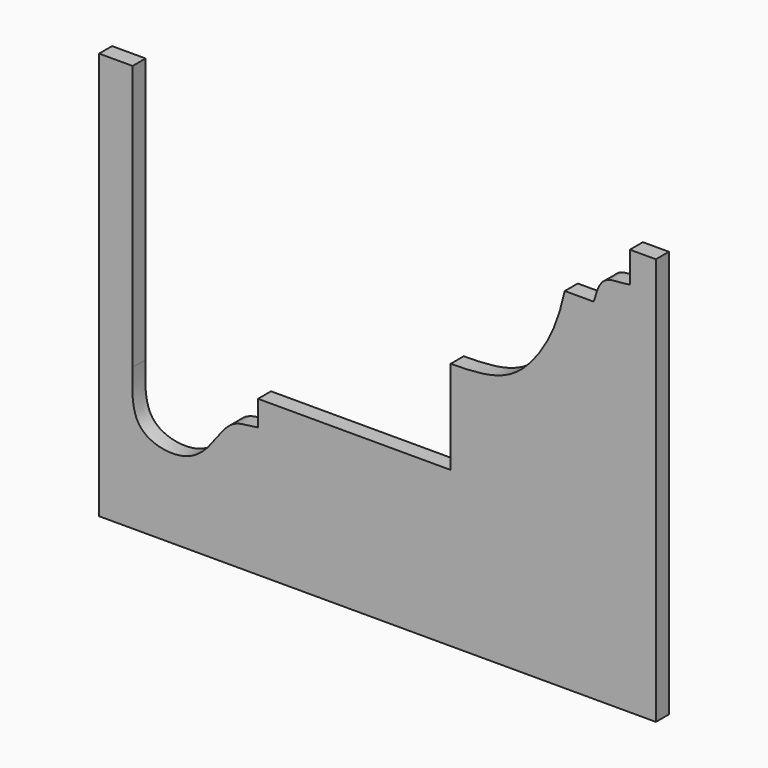
from build123d import *

# Parameters (mm, degrees)
F2_DEPTH = 10


with BuildPart() as f2:
    # F1 (on face) → F2 (new body)
    with BuildSketch(Plane.XZ):
        with BuildLine():
            Line((-91.9840037823, -31.2996767461), (-91.9840037823, 131.8993419409))
            Line((-91.9840037823, 131.8993419409), (-112.6081570983, 131.8993419409))
            Line((-112.6081570983, 131.8993419409), (-112.6081570983, -118.7344565988))
            Line((-112.6081570983, -118.7344565988), (230.0193011761, -118.7344565988))
            Line((230.0193011761, -118.7344565988), (230.0193011761, 131.8993419409))
            Line((230.0193011761, 131.8993419409), (214.0238434076, 131.8993419409))
            Line((214.0238434076, 131.8993419409), (214.0238434076, 113.0083352327))
            add(Edge.make_bspline(
                [(191.6237324476, 96.4869484305), (192.4980250224, 98.1278702864), (193.1536069546, 101.9439997116), (196.1146778047, 108.6562828707), (201.6165341433, 112.5583739062), (211.8606585251, 112.2793213926), (214.0238434076, 113.0083352327)],
                knots=[0, 0, 0, 0, 0.2157210018, 0.4532431975, 0.6893360054, 1, 1, 1, 1], degree=3))
            Line((191.6237324476, 96.4869484305), (173.9649176598, 96.4869484305))
            add(Edge.make_bspline(
                [(173.9649176598, 96.4869484305), (172.0666621983, 87.7106344295), (166.200808661, 67.3071544762), (145.3206230123, 39.4041475495), (121.2131008193, 34.3114486831), (109.1523088398, 34.3117546192), (103.772804141, 34.2541225255)],
                knots=[0, 0, 0, 0, 0.2707270162, 0.5572229358, 0.7957939194, 1, 1, 1, 1], degree=3))
            Line((103.772804141, 34.2541225255), (103.772804141, -23.3063530177))
            Line((103.772804141, -23.3063530177), (-14.8291196674, -23.3063530177))
            Line((-14.8291196674, -23.3063530177), (-14.8291196674, -38.8501137495))
            add(Edge.make_bspline(
                [(-14.8291196674, -38.8501137495), (-19.5772007963, -39.8984086665), (-31.9000289258, -38.8742055052), (-43.0777025398, -58.4234253449), (-59.6611048278, -73.1198238571), (-94.1107291621, -66.6840596527), (-92.2154498937, -41.7158947129), (-91.9840037823, -31.2996767461)],
                knots=[0, 0, 0, 0, 0.1643265607, 0.3546135647, 0.5490488256, 0.7659434096, 1, 1, 1, 1], degree=3))
        make_face()
    extrude(amount=F2_DEPTH)


solid = f2.part
